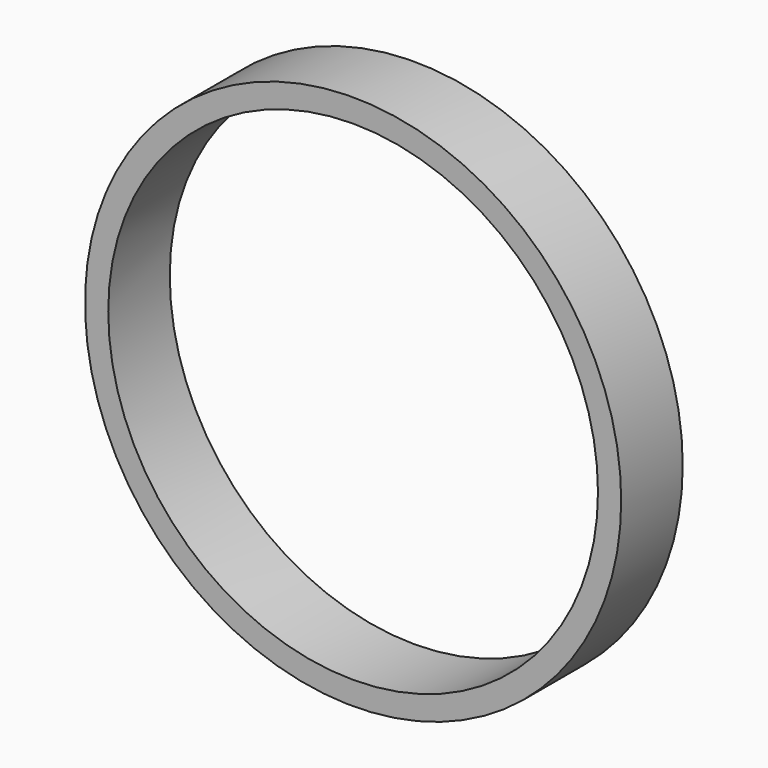
from build123d import *

# Parameters (mm, degrees)
F0_R     = 44.275413932
F1_DEPTH = 6.35


# Not quite as in the source:
# - the program builds the solid bodies; features that only make, move or delete a surface that nothing else refers to are left out


with BuildPart() as f1:
    # F0 (on Front) → F1 (new body, symmetric)
    with BuildSketch(Plane.XZ):
        Circle(F0_R)
        with BuildLine():
            ThreePointArc((-40.4384616778, 0), (0, 40.4384616778), (40.4384616778, 0))
            ThreePointArc((40.4384616778, 0), (0, -40.4384616778), (-40.4384616778, 0))
        make_face(mode=Mode.SUBTRACT)
    extrude(amount=F1_DEPTH, both=True)


solid = f1.part
